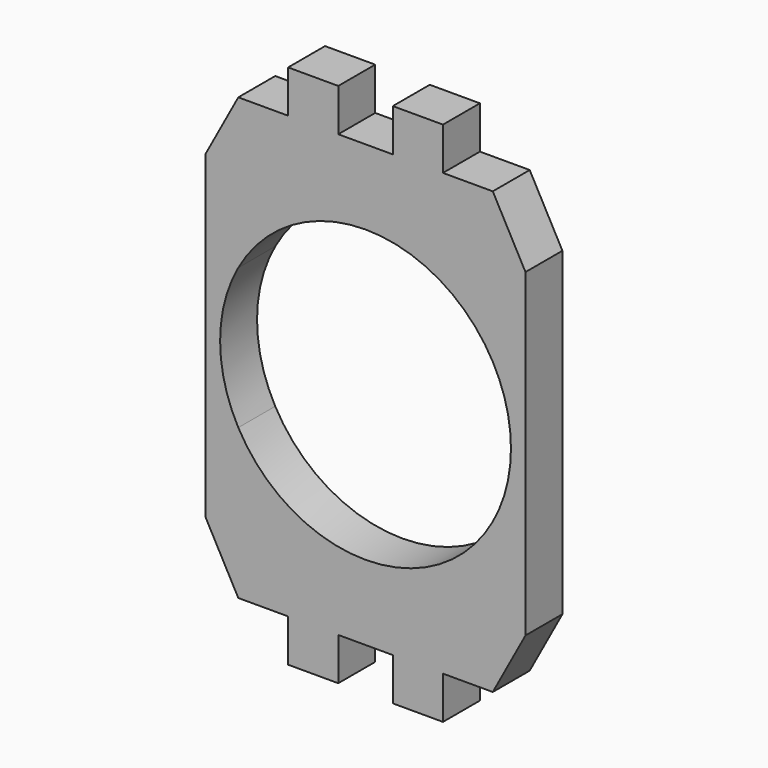
from build123d import *

# Parameters (mm, degrees)
F0_W     = 35
F0_H     = 8.31089
F1_DEPTH = 6.35
F2_W     = 6.9
F2_H     = 5.85
F3_DEPTH = 6.35


# Not quite as in the source:
# - a length typed as a fraction of an inch, garbled in the dataset ("3 / 203.2 mm" for 3/8 in), is restored


with BuildPart() as f1:
    # F0 (on Front) → F1 (new body)
    with BuildSketch(Plane.XZ):
        with BuildLine():
            ThreePointArc((17.5, 9.6824583655), (19.364916731, 5), (20, 0))
            ThreePointArc((20, 0), (19.364916731, -5), (17.5, -9.6824583655))
            Line((17.5, -9.6824583655), (17.5, -22))
            Line((17.5, -22), (22, -22))
            Line((22, -22), (22, 22))
            Line((22, 22), (17.5, 22))
            Line((17.5, 22), (17.5, 9.6824583655))
        make_face()
        with BuildLine():
            ThreePointArc((-17.5, -9.6824583655), (-20, 0), (-17.5, 9.6824583655))
            Line((-17.5, 9.6824583655), (-17.5, 22))
            Line((-17.5, 22), (-22, 22))
            Line((-22, 22), (-22, -22))
            Line((-22, -22), (-17.5, -22))
            Line((-17.5, -22), (-17.5, -9.6824583655))
        make_face()
        with Locations((0, 26.155445)):
            Rectangle(F0_W, F0_H)
        Polygon((17.5, 30.31089), (17.5, 22), (22, 22), align=None)
        Polygon((22, -22), (17.5, -22), (17.5, -30.31089), align=None)
        with Locations((0, -26.155445)):
            Rectangle(F0_W, F0_H)
        Polygon((-22, 22), (-17.5, 22), (-17.5, 30.31089), align=None)
        Polygon((-17.5, -30.31089), (-17.5, -22), (-22, -22), align=None)
        with BuildLine():
            ThreePointArc((-17.5, 9.6824583655), (0, 20), (17.5, 9.6824583655))
            Line((17.5, 9.6824583655), (17.5, 22))
            Line((17.5, 22), (-17.5, 22))
            Line((-17.5, 22), (-17.5, 9.6824583655))
        make_face()
        with BuildLine():
            Line((17.5, -22), (17.5, -9.6824583655))
            ThreePointArc((17.5, -9.6824583655), (0, -20), (-17.5, -9.6824583655))
            Line((-17.5, -9.6824583655), (-17.5, -22))
            Line((-17.5, -22), (17.5, -22))
        make_face()
    extrude(amount=F1_DEPTH)

    # F2 (on face) → F3 (join)
    with BuildSketch(Plane.XZ.offset(6.35)):
        with Locations((-7.2, 33.23589)):
            Rectangle(F2_W, F2_H)
        with Locations((7.2, 33.23589)):
            Rectangle(F2_W, F2_H)
        with Locations((-7.2, -33.23589)):
            Rectangle(F2_W, F2_H)
        with Locations((7.2, -33.23589)):
            Rectangle(F2_W, F2_H)
    extrude(amount=-F3_DEPTH)


solid = f1.part
